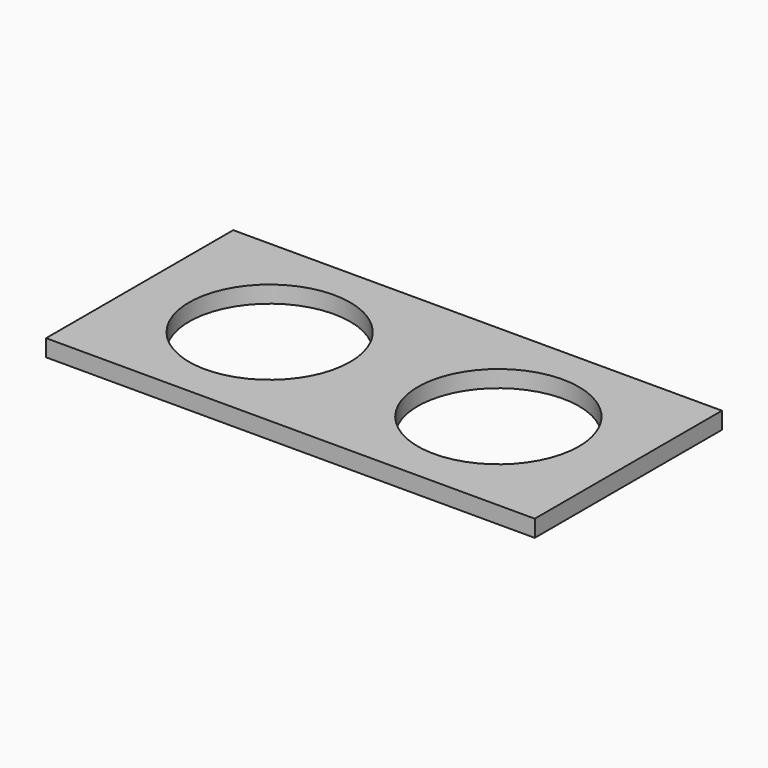
from build123d import *

# Parameters (mm, degrees)
F0_W     = 596.9
F0_H     = 285.75
F0_R     = 98.425
F1_DEPTH = 20.6375


# Not quite as in the source:
# - a length typed as a fraction of an inch, garbled in the dataset ("3 / 203.2 mm" for 3/8 in), is restored


with BuildPart() as f1:
    # F0 (on Top) → F1 (new body)
    with BuildSketch(Plane.XY):
        Rectangle(F0_W, F0_H)
        with Locations((-139.7, 0)):
            Circle(F0_R, mode=Mode.SUBTRACT)
        with Locations((139.7, 0)):
            Circle(F0_R, mode=Mode.SUBTRACT)
    extrude(amount=F1_DEPTH)


solid = f1.part
